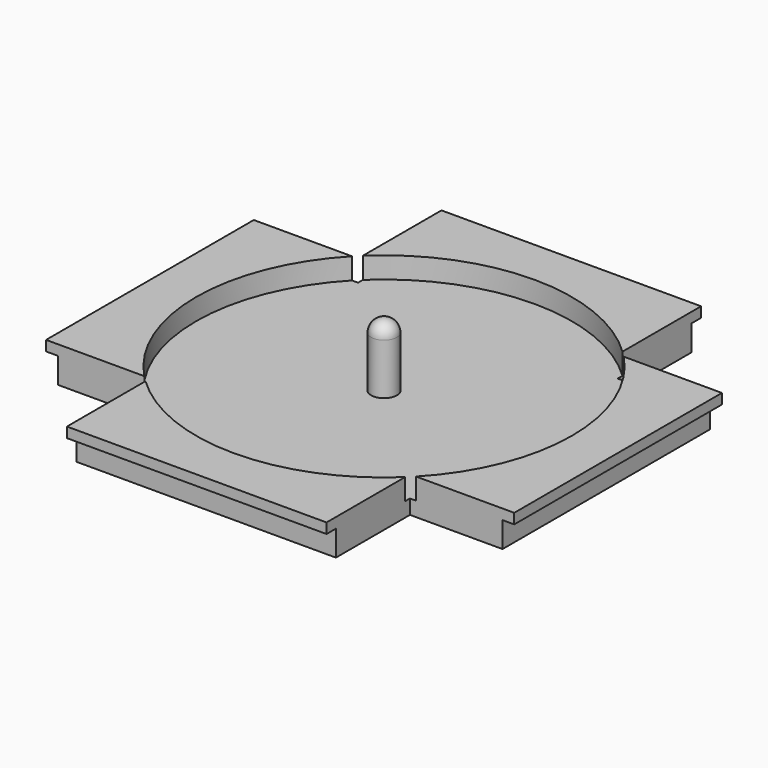
from build123d import *

# Parameters (mm, degrees)
F0_W             = 104.5
F0_H             = 104.5
F1_DEPTH         = 6
F2_W             = 110
F2_H             = 110
F2_W_2           = 104.5
F2_H_2           = 104.5
F3_DEPTH         = 2.4
F4_R             = 3.025
F5_DEPTH         = 10
F6_R             = 44.15
F6_R_2           = 3.025
F7_DEPTH         = 5
F8_R             = 3
F10_DEPTH        = 8.401
F10_COPIES_COUNT = 4


# Not quite as in the source:
# - a pattern or mirror of a feature is missing from the dataset's text; its kind, count and spacing are read off the source's solid


with BuildPart() as f1:
    # F0 (on Top) → F1 (new body)
    with BuildSketch(Plane.XY):
        Rectangle(F0_W, F0_H)
    extrude(amount=F1_DEPTH)

    # F2 (on face) → F3 (join)
    with BuildSketch(Plane.XY.offset(6)):
        Rectangle(F2_W, F2_H)
        Rectangle(F2_W_2, F2_H_2, mode=Mode.SUBTRACT)
        Rectangle(F2_W_2, F2_H_2)
    extrude(amount=F3_DEPTH)

    # F4 (on face) → F5 (join)
    with BuildSketch(Plane.XY.offset(8.4)):
        Circle(F4_R)
    extrude(amount=F5_DEPTH)

    # F6 (on face) → F7 (cut)
    with BuildSketch(Plane.XY.offset(8.4)):
        Circle(F6_R)
        Circle(F6_R_2, mode=Mode.SUBTRACT)
    extrude(amount=-F7_DEPTH, mode=Mode.SUBTRACT)

    # F8
    f8_edges = [f1.edges().sort_by_distance(p)[0] for p in [
        (-3.025, 0, 18.4),
    ]]
    fillet(f8_edges, radius=F8_R)

    # F9 (on face) → F10 (cut, through all)
    with BuildSketch(Plane.XY.offset(8.4)):
        with BuildLine():
            Line((-30.5, 31.9213486557), (-30.5, 55))
            Line((-30.5, 55), (-55, 55))
            Line((-55, 55), (-55, 30.5))
            Line((-55, 30.5), (-31.9213486557, 30.5))
            ThreePointArc((-31.9213486557, 30.5), (-31.2187643894, 31.2187643894), (-30.5, 31.9213486557))
        make_face()
        with BuildLine():
            Line((-30.5, 30.5), (-30.5, 31.9213486557))
            ThreePointArc((-30.5, 31.9213486557), (-31.2187643894, 31.2187643894), (-31.9213486557, 30.5))
            Line((-31.9213486557, 30.5), (-30.5, 30.5))
        make_face()
    f10 = extrude(amount=-F10_DEPTH, mode=Mode.SUBTRACT)

    # F10_copies: F10 ×4 about axis
    f10_copies_axis = Axis((0, 0, 0), (0, 0, 1))
    for i in range(1, F10_COPIES_COUNT):
        add(f10.rotate(f10_copies_axis, i * 360 / F10_COPIES_COUNT), mode=Mode.SUBTRACT)


solid = f1.part
